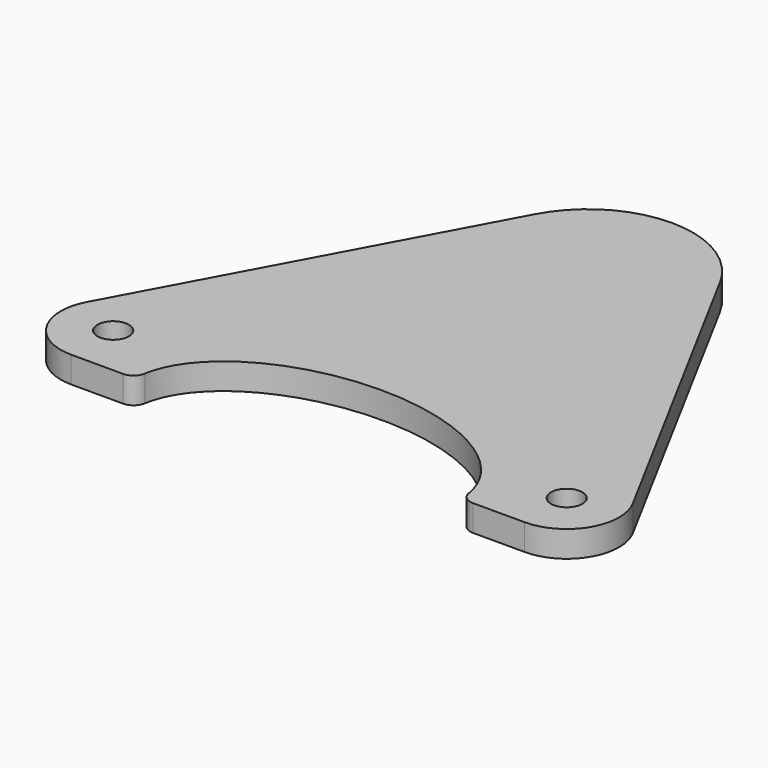
from build123d import *

# Parameters (mm, degrees)
F1_DEPTH = 10
F3_D     = 12
F5_DEPTH = 25
F6_R     = 5


# Not quite as in the source:
# - a pattern or mirror of a feature is missing from the dataset's text; its kind, count and spacing are read off the source's solid


with BuildPart() as f1:
    # F0 (on Top) → F1 (new body)
    with BuildSketch(Plane.XY):
        with BuildLine():
            Line((-86.4857615178, 0), (0, 0))
            Line((0, 0), (86.4857615178, 0))
            ThreePointArc((86.4857615178, 0), (103.6601107493, 9.7510132951), (104.0877292116, 29.4958271523))
            Line((104.0877292116, 29.4958271523), (35.2039353876, 157.1824724621))
            ThreePointArc((35.2039353876, 157.1824724621), (0, 178.1908181575), (-35.2039353876, 157.1824724621))
            Line((-35.2039353876, 157.1824724621), (-104.0877292116, 29.4958271523))
            ThreePointArc((-104.0877292116, 29.4958271523), (-103.6601107493, 9.7510132951), (-86.4857615178, 0))
        make_face()
    extrude(amount=F1_DEPTH)

    # F3 (through all)
    with Locations(Plane.XY.offset(10)):
        with Locations((86.4857615178, 20)):
            f3 = Hole(F3_D / 2)

    # F3_copies: F3 across plane
    add(f3.mirror(Plane(origin=(0, 0, 0), x_dir=(0, 0, -1), z_dir=(-1, 0, 0))), mode=Mode.SUBTRACT)

    # F4 (on face) → F5 (cut)
    with BuildSketch(Plane.XY.offset(10)):
        with BuildLine():
            add(Edge.make_bspline(
                [(62.1145702899, 0), (62.1145702899, 69.1070951712), (-31.0572851449, 34.5535475856), (-124.2291405797, 0), (-31.0572851449, -34.5535475856), (62.1145702899, -69.1070951712), (62.1145702899, 0)],
                knots=[0, 0, 0, 2.0943951024, 2.0943951024, 4.1887902048, 4.1887902048, 6.2831853072, 6.2831853072, 6.2831853072], degree=2, weights=[1, 0.5, 1, 0.5, 1, 0.5, 1]))
        make_face()
    extrude(amount=-F5_DEPTH, mode=Mode.SUBTRACT)

    # F6
    f6_edges = [f1.edges().sort_by_distance(p)[0] for p in [
        (-62.11457, 0, 5),
        (62.11457, 0, 5),
    ]]
    fillet(f6_edges, radius=F6_R)


solid = f1.part
